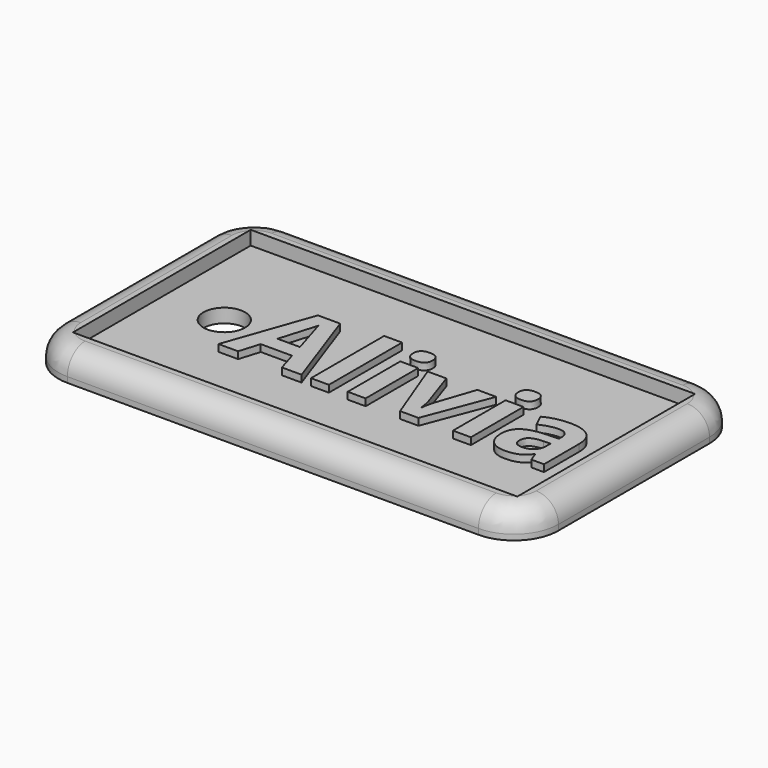
from build123d import *

# Parameters (mm, degrees)
F0_W         = 50.8
F0_H         = 25.4
F0_R         = 2.38125
F1_DEPTH     = 1.5875
F0_W_2       = 57.15
F0_H_2       = 31.75
F2_DEPTH     = 3.175
F3_R         = 5.08
F4_T1_DEPTH  = 46.99
F4_T3_DEPTH  = 21.59
F4_T6_ANGLE  = 90
F4_T8_ANGLE  = 90
F4_T10_ANGLE = 90
F4_T12_ANGLE = 90
F6_TEXT_SIZE = 13.7646062659
F7_DEPTH     = 0.79375


# Not quite as in the source:
# - a fillet or chamfer that OpenCascade refuses, or shapes differently, is made with other operations: its cross-section is extruded or revolved along the edge and cut away or added
# - Text() gives the source's letters only with a copy of the font that has no kerning and outlines rounded to 1/6400 em; it was checked with that copy


with BuildPart() as f1:
    # F0 (on Top) → F1 (new body)
    with BuildSketch(Plane.XY):
        with Locations((25.4, 12.7)):
            Rectangle(F0_W, F0_H)
        with Locations((7.14375, 12.7)):
            Circle(F0_R, mode=Mode.SUBTRACT)
    extrude(amount=F1_DEPTH)

    # F0 (on Top) → F2 (join)
    with BuildSketch(Plane.XY):
        with Locations((25.4, 12.7)):
            Rectangle(F0_W_2, F0_H_2)
        with Locations((25.4, 12.7)):
            Rectangle(F0_W, F0_H, mode=Mode.SUBTRACT)
    extrude(amount=F2_DEPTH)

    # F3
    f3_edges = [f1.edges().sort_by_distance(p)[0] for p in [
        (53.975, -3.175, 1.5875),
        (-3.175, -3.175, 1.5875),
        (53.975, 28.575, 1.5875),
        (-3.175, 28.575, 1.5875),
    ]]
    fillet(f3_edges, radius=F3_R)

    # F4: fillet of radius 2.54 on 8 edges, made by hand

    # F4_s2 → F4_t1 (cut)
    with BuildSketch(Plane.YZ.offset(1.905)):
        with BuildLine():
            ThreePointArc((-3.175, 0.635), (-2.4310512242, 2.4310512242), (-0.635, 3.175))
            Line((-0.635, 3.175), (-3.175, 3.175))
            Line((-3.175, 3.175), (-3.175, 0.635))
        make_face()
        with BuildLine():
            ThreePointArc((28.575, 0.635), (27.8310512242, 2.4310512242), (26.035, 3.175))
            Line((26.035, 3.175), (28.575, 3.175))
            Line((28.575, 3.175), (28.575, 0.635))
        make_face()
    extrude(amount=F4_T1_DEPTH, mode=Mode.SUBTRACT)

    # F4_s4 → F4_t3 (cut)
    with BuildSketch(Plane.XZ.offset(-23.495)):
        with BuildLine():
            ThreePointArc((53.975, 0.635), (53.2310512242, 2.4310512242), (51.435, 3.175))
            Line((51.435, 3.175), (53.975, 3.175))
            Line((53.975, 3.175), (53.975, 0.635))
        make_face()
        with BuildLine():
            ThreePointArc((-3.175, 0.635), (-2.4310512242, 2.4310512242), (-0.635, 3.175))
            Line((-0.635, 3.175), (-3.175, 3.175))
            Line((-3.175, 3.175), (-3.175, 0.635))
        make_face()
    extrude(amount=F4_T3_DEPTH, mode=Mode.SUBTRACT)

    # F4_s5 → F4_t6 (revolve, cut)
    with BuildSketch(Plane.YZ.offset(48.895)):
        with BuildLine():
            ThreePointArc((28.575, 0.635), (27.8310512242, 2.4310512242), (26.035, 3.175))
            Line((26.035, 3.175), (28.575, 3.175))
            Line((28.575, 3.175), (28.575, 0.635))
        make_face()
    revolve(axis=Axis((48.895, 23.495, 3.175), (0, 0, -1)), revolution_arc=F4_T6_ANGLE, mode=Mode.SUBTRACT)

    # F4_s7 → F4_t8 (revolve, cut)
    with BuildSketch(Plane.YZ.offset(1.905)):
        with BuildLine():
            ThreePointArc((28.575, 0.635), (27.8310512242, 2.4310512242), (26.035, 3.175))
            Line((26.035, 3.175), (28.575, 3.175))
            Line((28.575, 3.175), (28.575, 0.635))
        make_face()
    revolve(axis=Axis((1.905, 23.495, 3.175), (0, 0, 1)), revolution_arc=F4_T8_ANGLE, mode=Mode.SUBTRACT)

    # F4_s9 → F4_t10 (revolve, cut)
    with BuildSketch(Plane.YZ.offset(48.895)):
        with BuildLine():
            ThreePointArc((-3.175, 0.635), (-2.4310512242, 2.4310512242), (-0.635, 3.175))
            Line((-0.635, 3.175), (-3.175, 3.175))
            Line((-3.175, 3.175), (-3.175, 0.635))
        make_face()
    revolve(axis=Axis((48.895, 1.905, 3.175), (0, 0, 1)), revolution_arc=F4_T10_ANGLE, mode=Mode.SUBTRACT)

    # F4_s11 → F4_t12 (revolve, cut)
    with BuildSketch(Plane.XZ.offset(-1.905)):
        with BuildLine():
            ThreePointArc((-3.175, 0.635), (-2.4310512242, 2.4310512242), (-0.635, 3.175))
            Line((-0.635, 3.175), (-3.175, 3.175))
            Line((-3.175, 3.175), (-3.175, 0.635))
        make_face()
    revolve(axis=Axis((1.905, 1.905, 3.175), (0, 0, 1)), revolution_arc=F4_T12_ANGLE, mode=Mode.SUBTRACT)

    # F6 (on face) → F7 (join)
    with BuildSketch(Plane.XY.offset(1.5875)):
        with Locations((10.5955184053, 7.5530806017)):
            Text('Alivia', F6_TEXT_SIZE, font='Open Sans', font_style=FontStyle.BOLD, text_align=(TextAlign.LEFT, TextAlign.BOTTOM))
    extrude(amount=F7_DEPTH)


solid = f1.part
